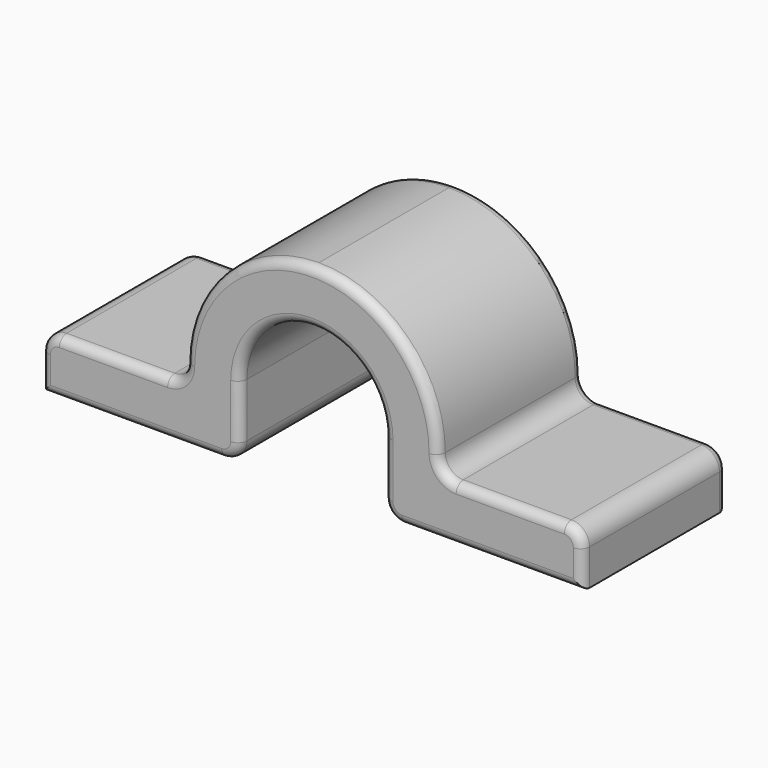
from build123d import *

# Parameters (mm, degrees)
F1_DEPTH     = 10
F2_R         = 0.99999
F3_T1_DEPTH  = 1e-05
F3_T3_DEPTH  = 3.00001
F3_T5_DEPTH  = 11.25001
F3_T7_DEPTH  = 6.00002
F3_T9_DEPTH  = 3.25001
F3_T12_ANGLE = 107.9121236547
F3_T14_ANGLE = 100.2354992312
F3_T16_ANGLE = 90
F3_T18_ANGLE = 107.9121236547
F3_T20_ANGLE = 90
F3_T22_ANGLE = 100.2354992312
F3_T24_ANGLE = 90
F3_T26_ANGLE = 90
F3_T28_ANGLE = 90
F3_T30_ANGLE = 90


# Not quite as in the source:
# - a fillet or chamfer that OpenCascade refuses, or shapes differently, is made with other operations: its cross-section is extruded or revolved along the edge and cut away or added
# - a fillet or chamfer is up to 0.001 mm smaller than in the source, because OpenCascade refuses the exact size


with BuildPart() as f1:
    # F0 (on Front) → F1 (new body)
    with BuildSketch(Plane.XZ):
        with BuildLine():
            Line((7, 3), (7, 4))
            ThreePointArc((7, 4), (6.6787700412, 1.9038056538), (5.7445626465, 0))
            Line((5.7445626465, 0), (7, 0))
            Line((7, 0), (15, 0))
            Line((15, 0), (15, 3))
            Line((15, 3), (7, 3))
        make_face()
        with BuildLine():
            Line((7, 4), (4, 4))
            Line((4, 4), (4, 0))
            Line((4, 0), (5.7445626465, 0))
            ThreePointArc((5.7445626465, 0), (6.6787700412, 1.9038056538), (7, 4))
        make_face()
        with BuildLine():
            Line((0, 11), (0, 8))
            ThreePointArc((0, 8), (2.8284271247, 6.8284271247), (4, 4))
            Line((4, 4), (7, 4))
            ThreePointArc((7, 4), (4.9497474683, 8.9497474683), (0, 11))
        make_face()
    extrude(amount=F1_DEPTH)

    # F2 (radius 1 in the source; OpenCascade refuses exactly that, so slightly less here)
    f2_edges = [f1.edges().sort_by_distance(p)[0] for p in [
        (7, -5, 3),
        (4, -5, 0),
        (15, -5, 3),
    ]]
    fillet(f2_edges, radius=F2_R)

    # F3: fillet of radius 0.5 on 5 edges, made by hand

    # F3_s2 → F3_t1 (cut)
    with BuildSketch(Plane.XY.offset(3.99999)):
        with BuildLine():
            ThreePointArc((6.5, -10), (6.8535533906, -9.8535533906), (7, -9.5))
            Line((7, -9.5), (7, -10))
            Line((7, -10), (6.5, -10))
        make_face()
        with BuildLine():
            ThreePointArc((6.5, 0), (6.8535533906, -0.1464466094), (7, -0.5))
            Line((7, -0.5), (7, 0))
            Line((7, 0), (6.5, 0))
        make_face()
    extrude(amount=F3_T1_DEPTH, mode=Mode.SUBTRACT)

    # F3_s4 → F3_t3 (cut)
    with BuildSketch(Plane.XY.offset(0.99999)):
        with BuildLine():
            ThreePointArc((4.5, 0), (4.1464466094, -0.1464466094), (4, -0.5))
            Line((4, -0.5), (4, 0))
            Line((4, 0), (4.5, 0))
        make_face()
        with BuildLine():
            ThreePointArc((4.5, -10), (4.1464466094, -9.8535533906), (4, -9.5))
            Line((4, -9.5), (4, -10))
            Line((4, -10), (4.5, -10))
        make_face()
    extrude(amount=F3_T3_DEPTH, mode=Mode.SUBTRACT)

    # F3_s6 → F3_t5 (cut)
    with BuildSketch(Plane.YZ.offset(4.99999)):
        with BuildLine():
            ThreePointArc((0, 0.5), (-0.1464466094, 0.1464466094), (-0.5, 0))
            Line((-0.5, 0), (0, 0))
            Line((0, 0), (0, 0.5))
        make_face()
        with BuildLine():
            ThreePointArc((-9.5, 0), (-9.8535533906, 0.1464466094), (-10, 0.5))
            Line((-10, 0.5), (-10, 0))
            Line((-10, 0), (-9.5, 0))
        make_face()
    extrude(amount=F3_T5_DEPTH, mode=Mode.SUBTRACT)

    # F3_s8 → F3_t7 (cut)
    with BuildSketch(Plane.YZ.offset(7.99999)):
        with BuildLine():
            ThreePointArc((0, 2.5), (-0.1464466094, 2.8535533906), (-0.5, 3))
            Line((-0.5, 3), (0, 3))
            Line((0, 3), (0, 2.5))
        make_face()
        with BuildLine():
            ThreePointArc((-10, 2.5), (-9.8535533906, 2.8535533906), (-9.5, 3))
            Line((-9.5, 3), (-10, 3))
            Line((-10, 3), (-10, 2.5))
        make_face()
    extrude(amount=F3_T7_DEPTH, mode=Mode.SUBTRACT)

    # F3_s10 → F3_t9 (cut)
    with BuildSketch(Plane.XY.offset(-1.25)):
        with BuildLine():
            ThreePointArc((15, -0.5), (14.8535533906, -0.1464466094), (14.5, 0))
            Line((14.5, 0), (15, 0))
            Line((15, 0), (15, -0.5))
        make_face()
        with BuildLine():
            ThreePointArc((15, -9.5), (14.8535533906, -9.8535533906), (14.5, -10))
            Line((14.5, -10), (15, -10))
            Line((15, -10), (15, -9.5))
        make_face()
    extrude(amount=F3_T9_DEPTH, mode=Mode.SUBTRACT)

    # F3_s11 → F3_t12 (revolve, cut)
    with BuildSketch(Plane(origin=(1.1706017221, 0, 0.37836761), x_dir=(0, 1, 0), z_dir=(-0.9515293466, 0, -0.3075579661))):
        with BuildLine():
            ThreePointArc((-10, -8.3061173865), (-9.8535533906, -7.9525639959), (-9.5, -7.8061173865))
            Line((-9.5, -7.8061173865), (-10, -7.8061173865))
            Line((-10, -7.8061173865), (-10, -8.3061173865))
        make_face()
    revolve(axis=Axis((0, -10, 4), (0, 1, 0)), revolution_arc=F3_T12_ANGLE, mode=Mode.SUBTRACT)

    # F3_s13 → F3_t14 (revolve, cut)
    with BuildSketch(Plane.XY.offset(4)):
        with BuildLine():
            ThreePointArc((6.5, -10), (6.8535533906, -9.8535533906), (7, -9.5))
            Line((7, -9.5), (7, -10))
            Line((7, -10), (6.5, -10))
        make_face()
    revolve(axis=Axis((0, -10, 4), (0, -1, 0)), revolution_arc=F3_T14_ANGLE, mode=Mode.SUBTRACT)

    # F3_s15 → F3_t16 (revolve, cut)
    with BuildSketch(Plane.YZ.offset(7.99999)):
        with BuildLine():
            ThreePointArc((0, 2.5), (-0.1464466094, 2.8535533906), (-0.5, 3))
            Line((-0.5, 3), (0, 3))
            Line((0, 3), (0, 2.5))
        make_face()
    revolve(axis=Axis((7.99999, 0, 3.99999), (0, 1, 0)), revolution_arc=F3_T16_ANGLE, mode=Mode.SUBTRACT)

    # F3_s17 → F3_t18 (revolve, cut)
    with BuildSketch(Plane(origin=(1.1706017221, 0, 0.37836761), x_dir=(0, 1, 0), z_dir=(-0.9515293466, 0, -0.3075579661))):
        with BuildLine():
            ThreePointArc((0, -8.3061173865), (-0.1464466094, -7.9525639959), (-0.5, -7.8061173865))
            Line((-0.5, -7.8061173865), (0, -7.8061173865))
            Line((0, -7.8061173865), (0, -8.3061173865))
        make_face()
    revolve(axis=Axis((0, 0, 4), (0, 1, 0)), revolution_arc=F3_T18_ANGLE, mode=Mode.SUBTRACT)

    # F3_s19 → F3_t20 (revolve, cut)
    with BuildSketch(Plane.XY.offset(0.99999)):
        with BuildLine():
            ThreePointArc((4.5, 0), (4.1464466094, -0.1464466094), (4, -0.5))
            Line((4, -0.5), (4, 0))
            Line((4, 0), (4.5, 0))
        make_face()
    revolve(axis=Axis((4.99999, 0, 0.99999), (0, -1, 0)), revolution_arc=F3_T20_ANGLE, mode=Mode.SUBTRACT)

    # F3_s21 → F3_t22 (revolve, cut)
    with BuildSketch(Plane.XY.offset(4)):
        with BuildLine():
            ThreePointArc((6.5, 0), (6.8535533906, -0.1464466094), (7, -0.5))
            Line((7, -0.5), (7, 0))
            Line((7, 0), (6.5, 0))
        make_face()
    revolve(axis=Axis((0, 0, 4), (0, -1, 0)), revolution_arc=F3_T22_ANGLE, mode=Mode.SUBTRACT)

    # F3_s23 → F3_t24 (revolve, cut)
    with BuildSketch(Plane.XY.offset(2.00001)):
        with BuildLine():
            ThreePointArc((14.5, 0), (14.8535533906, -0.1464466094), (15, -0.5))
            Line((15, -0.5), (15, 0))
            Line((15, 0), (14.5, 0))
        make_face()
    revolve(axis=Axis((14.00001, 0, 2.00001), (0, -1, 0)), revolution_arc=F3_T24_ANGLE, mode=Mode.SUBTRACT)

    # F3_s25 → F3_t26 (revolve, cut)
    with BuildSketch(Plane.YZ.offset(7.99999)):
        with BuildLine():
            ThreePointArc((-10, 2.5), (-9.8535533906, 2.8535533906), (-9.5, 3))
            Line((-9.5, 3), (-10, 3))
            Line((-10, 3), (-10, 2.5))
        make_face()
    revolve(axis=Axis((7.99999, -10, 3.99999), (0, 1, 0)), revolution_arc=F3_T26_ANGLE, mode=Mode.SUBTRACT)

    # F3_s27 → F3_t28 (revolve, cut)
    with BuildSketch(Plane.XY.offset(2.00001)):
        with BuildLine():
            ThreePointArc((15, -9.5), (14.8535533906, -9.8535533906), (14.5, -10))
            Line((14.5, -10), (15, -10))
            Line((15, -10), (15, -9.5))
        make_face()
    revolve(axis=Axis((14.00001, -10, 2.00001), (0, -1, 0)), revolution_arc=F3_T28_ANGLE, mode=Mode.SUBTRACT)

    # F3_s29 → F3_t30 (revolve, cut)
    with BuildSketch(Plane.XY.offset(0.99999)):
        with BuildLine():
            ThreePointArc((4.5, -10), (4.1464466094, -9.8535533906), (4, -9.5))
            Line((4, -9.5), (4, -10))
            Line((4, -10), (4.5, -10))
        make_face()
    revolve(axis=Axis((4.99999, -10, 0.99999), (0, -1, 0)), revolution_arc=F3_T30_ANGLE, mode=Mode.SUBTRACT)

    # F4: F1 across face


with BuildPart() as f1_1:
    add(f1.part)
    add(f1.part.mirror(Plane(origin=(0, -5, 9.5), x_dir=(0, -1, 0), z_dir=(-1, 0, 0))))


solid = f1_1.part
